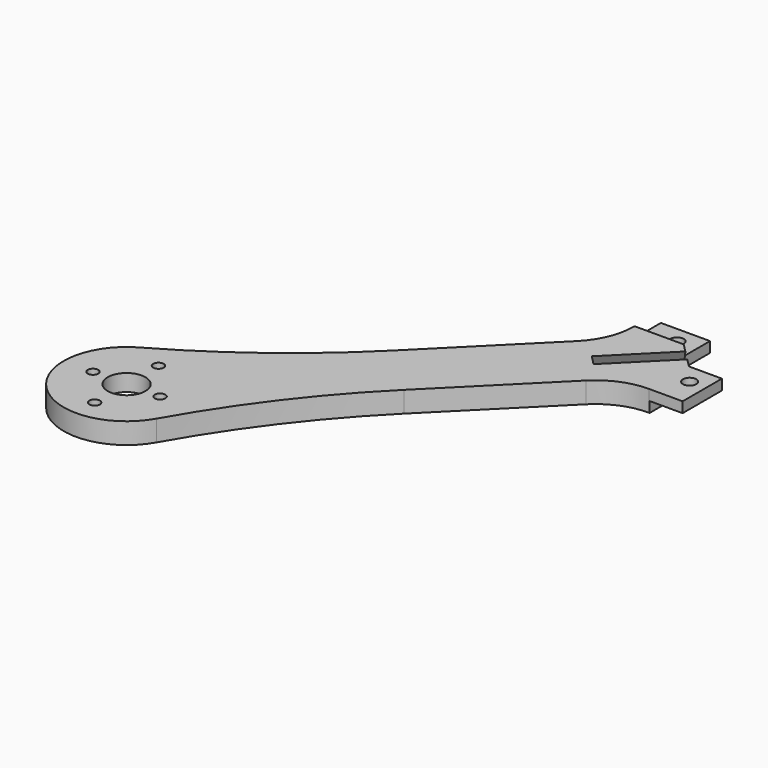
from build123d import *

# Parameters (mm, degrees)
F0_R     = 1.25
F0_R_2   = 4.5
F1_DEPTH = 5
F0_W     = 11.7265549134
F0_H     = 7.858
F0_R_3   = 1.6
F2_DEPTH = 2.5
F0_W_2   = 7.858
F0_H_2   = 11.7265549134
F3_DEPTH = 5
F4_DEPTH = 2.5
F5_DEPTH = 1
F6_R     = 175
F8_DEPTH = 25


# Not quite as in the source:
# - a feature names something its author has since deleted; it is built from what else it names


with BuildPart() as f1:
    # F0 (on Top) → F1 (new body)
    with BuildSketch(Plane.XY):
        with BuildLine():
            Line((-10.2734450866, -3.929), (-22, -3.929))
            Line((-22, -3.929), (-22, -4.058874503))
            ThreePointArc((-22, -4.058874503), (-23.2179274798, -10.1818094209), (-26.686291501, -15.372583002))
            Line((-26.686291501, -15.372583002), (-78.0019548635, -66.6882463645))
            ThreePointArc((-78.0019548635, -66.6882463645), (-91.9238815543, -91.9238815543), (-66.6882463645, -78.0019548635))
            Line((-66.6882463645, -78.0019548635), (-15.372583002, -26.686291501))
            ThreePointArc((-15.372583002, -26.686291501), (-10.1818094209, -23.2179274798), (-4.058874503, -22))
            Line((-4.058874503, -22), (-3.929, -22))
            Line((-3.929, -22), (-3.929, -10.2734450866))
            Line((-3.929, -10.2734450866), (-5.9698516934, -8.2325933932))
            Line((-5.9698516934, -8.2325933932), (-18.3937554159, -20.6564971157))
            Line((-18.3937554159, -20.6564971157), (-15.6360389693, -23.4142135624))
            ThreePointArc((-15.6360389693, -23.4142135624), (-15.3431457505, -24.1213203436), (-15.6360389693, -24.8284271247))
            Line((-15.6360389693, -24.8284271247), (-68.3544854934, -77.5468736488))
            ThreePointArc((-68.3544854934, -77.5468736488), (-90.8632213825, -90.8632213825), (-77.5468736488, -68.3544854934))
            Line((-77.5468736488, -68.3544854934), (-24.8284271247, -15.6360389693))
            ThreePointArc((-24.8284271247, -15.6360389693), (-24.1213203436, -15.3431457505), (-23.4142135624, -15.6360389693))
            Line((-23.4142135624, -15.6360389693), (-20.6564971157, -18.3937554159))
            Line((-20.6564971157, -18.3937554159), (-8.2325933932, -5.9698516934))
            Line((-8.2325933932, -5.9698516934), (-10.2734450866, -3.929))
        make_face()
        with BuildLine():
            Line((-18.3937554159, -20.6564971157), (-20.6564971157, -18.3937554159))
            Line((-20.6564971157, -18.3937554159), (-23.4142135624, -15.6360389693))
            ThreePointArc((-23.4142135624, -15.6360389693), (-24.1213203436, -15.3431457505), (-24.8284271247, -15.6360389693))
            Line((-24.8284271247, -15.6360389693), (-77.5468736488, -68.3544854934))
            ThreePointArc((-77.5468736488, -68.3544854934), (-90.8632213825, -90.8632213825), (-68.3544854934, -77.5468736488))
            Line((-68.3544854934, -77.5468736488), (-15.6360389693, -24.8284271247))
            ThreePointArc((-15.6360389693, -24.8284271247), (-15.3431457505, -24.1213203436), (-15.6360389693, -23.4142135624))
            Line((-15.6360389693, -23.4142135624), (-18.3937554159, -20.6564971157))
        make_face()
        with Locations((-81.3172798365, -90.8172798365)):
            Circle(F0_R, mode=Mode.SUBTRACT)
        with Locations((-89.3172798365, -81.3172798365)):
            Circle(F0_R, mode=Mode.SUBTRACT)
        with Locations((-81.3172798365, -81.3172798365)):
            Circle(F0_R_2, mode=Mode.SUBTRACT)
        with Locations((-73.3172798365, -81.3172798365)):
            Circle(F0_R, mode=Mode.SUBTRACT)
        with Locations((-81.3172798365, -71.8172798365)):
            Circle(F0_R, mode=Mode.SUBTRACT)
    extrude(amount=F1_DEPTH)

    # F0 (on Top) → F2 (join)
    with BuildSketch(Plane.XY):
        with Locations((-16.1367225433, 0)):
            Rectangle(F0_W, F0_H)
        with Locations((-15, 0)):
            Circle(F0_R_3, mode=Mode.SUBTRACT)
    extrude(amount=F2_DEPTH)

    # F0 (on Top) → F3 (join)
    with BuildSketch(Plane.XY):
        with Locations((0, -16.1367225433)):
            Rectangle(F0_W_2, F0_H_2)
        with Locations((0, -15)):
            Circle(F0_R_3, mode=Mode.SUBTRACT)
    extrude(amount=F3_DEPTH)

    # F0 (on Top) → F4 (cut)
    with BuildSketch(Plane.XY):
        with Locations((0, -16.1367225433)):
            Rectangle(F0_W_2, F0_H_2)
        with Locations((0, -15)):
            Circle(F0_R_3, mode=Mode.SUBTRACT)
    extrude(amount=F4_DEPTH, mode=Mode.SUBTRACT)

    # F0 (on Top) → F5 (cut)
    with BuildSketch(Plane.XY):
        with BuildLine():
            Line((-18.3937554159, -20.6564971157), (-20.6564971157, -18.3937554159))
            Line((-20.6564971157, -18.3937554159), (-23.4142135624, -15.6360389693))
            ThreePointArc((-23.4142135624, -15.6360389693), (-24.1213203436, -15.3431457505), (-24.8284271247, -15.6360389693))
            Line((-24.8284271247, -15.6360389693), (-77.5468736488, -68.3544854934))
            ThreePointArc((-77.5468736488, -68.3544854934), (-90.8632213825, -90.8632213825), (-68.3544854934, -77.5468736488))
            Line((-68.3544854934, -77.5468736488), (-15.6360389693, -24.8284271247))
            ThreePointArc((-15.6360389693, -24.8284271247), (-15.3431457505, -24.1213203436), (-15.6360389693, -23.4142135624))
            Line((-15.6360389693, -23.4142135624), (-18.3937554159, -20.6564971157))
        make_face()
        with Locations((-81.3172798365, -90.8172798365)):
            Circle(F0_R, mode=Mode.SUBTRACT)
        with Locations((-89.3172798365, -81.3172798365)):
            Circle(F0_R, mode=Mode.SUBTRACT)
        with Locations((-81.3172798365, -81.3172798365)):
            Circle(F0_R_2, mode=Mode.SUBTRACT)
        with Locations((-73.3172798365, -81.3172798365)):
            Circle(F0_R, mode=Mode.SUBTRACT)
        with Locations((-81.3172798365, -71.8172798365)):
            Circle(F0_R, mode=Mode.SUBTRACT)
    extrude(amount=F5_DEPTH, mode=Mode.SUBTRACT)

    # F6
    f6_edges = [f1.edges().sort_by_distance(p)[0] for p in [
        (-66.688246, -78.001955, 2.5),
        (-78.001955, -66.688246, 2.5),
    ]]
    fillet(f6_edges, radius=F6_R)

    # F7 (on face) → F8 (cut)
    with BuildSketch(Plane(origin=(-19.5251262658, -19.5251262658, 0), x_dir=(-0.7071067812, 0.7071067812, 0), z_dir=(0.7071067812, 0.7071067812, 0))):
        Polygon((4.4867513459, 0), (1.6, 5), (1.6, 1), (-1.6, 1), (-1.6, 5), (-4.4867513459, 0), align=None)
    extrude(amount=F8_DEPTH, mode=Mode.SUBTRACT)


solid = f1.part
